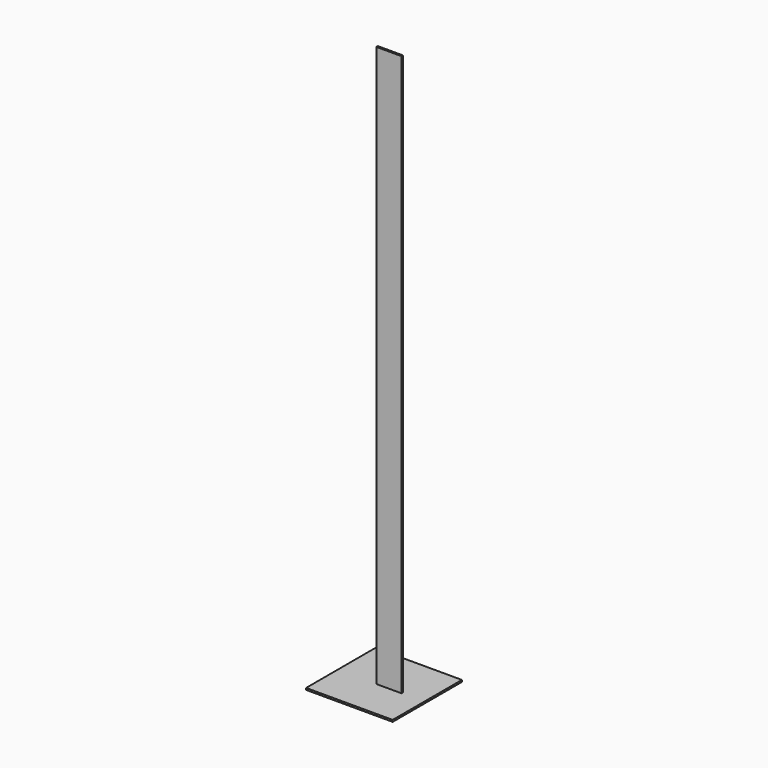
from build123d import *

# Parameters (mm, degrees)
F0_W     = 304.8
F0_H     = 304.8
F1_DEPTH = 6.35
F2_W     = 88.9
F2_H     = 6.35
F3_DEPTH = 1981.2


# Not quite as in the source:
# - a length typed as a fraction of an inch, garbled in the dataset ("3 / 203.2 mm" for 3/8 in), is restored


with BuildPart() as f1:
    # F0 (on Top) → F1 (new body)
    with BuildSketch(Plane.XY):
        with Locations((-48.9288084209, 3.6240073187)):
            Rectangle(F0_W, F0_H)
    extrude(amount=F1_DEPTH)

    # F2 (on Top) → F3 (join)
    with BuildSketch(Plane.XY):
        with Locations((-20.2900925651, -6.9411601371)):
            Rectangle(F2_W, F2_H)
    extrude(amount=F3_DEPTH)


solid = f1.part
